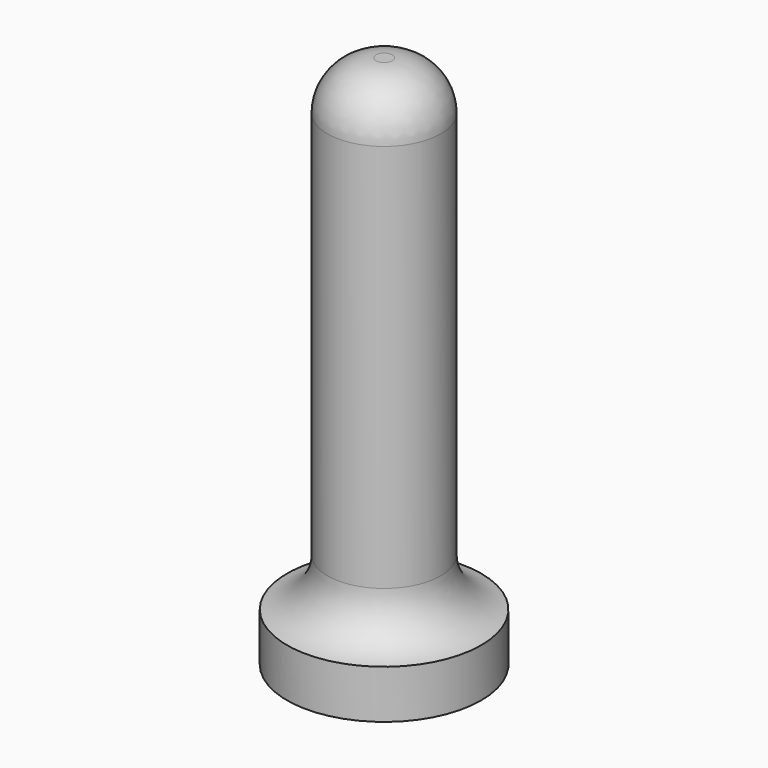
from build123d import *

# Parameters (mm, degrees)
F0_R     = 6
F1_DEPTH = 3
F2_R     = 3.5
F3_DEPTH = 30


# Not quite as in the source:
# - a fillet or chamfer that OpenCascade refuses, or shapes differently, is made with other operations: its cross-section is extruded or revolved along the edge and cut away or added


with BuildPart() as f1:
    # F0 (on Top) → F1 (new body)
    with BuildSketch(Plane.XY):
        Circle(F0_R)
    extrude(amount=F1_DEPTH)

    # F2 (on face) → F3 (join)
    with BuildSketch(Plane.XY.offset(3)):
        Circle(F2_R)
    extrude(amount=F3_DEPTH)

    # F4: fillet of radius 3 on 2 edges, made by hand

    # F4_s1 → F4_t2 (revolve)
    with BuildSketch(Plane.XZ):
        with BuildLine():
            ThreePointArc((6, 3), (4.2087121525, 4.0215482184), (3.5, 5.9580398916))
            Line((3.5, 5.9580398916), (3.5, 3))
            Line((3.5, 3), (6, 3))
        make_face()
    revolve(axis=Axis((0, 0, 3), (0, 0, 1)))

    # F4_s3 → F4_t4 (revolve, cut)
    with BuildSketch(Plane.XZ):
        with BuildLine():
            ThreePointArc((3.5, 30), (2.6213203436, 32.1213203436), (0.5, 33))
            Line((0.5, 33), (3.5, 33))
            Line((3.5, 33), (3.5, 30))
        make_face()
    revolve(axis=Axis((0, 0, 33), (0, 0, 1)), mode=Mode.SUBTRACT)


solid = f1.part
